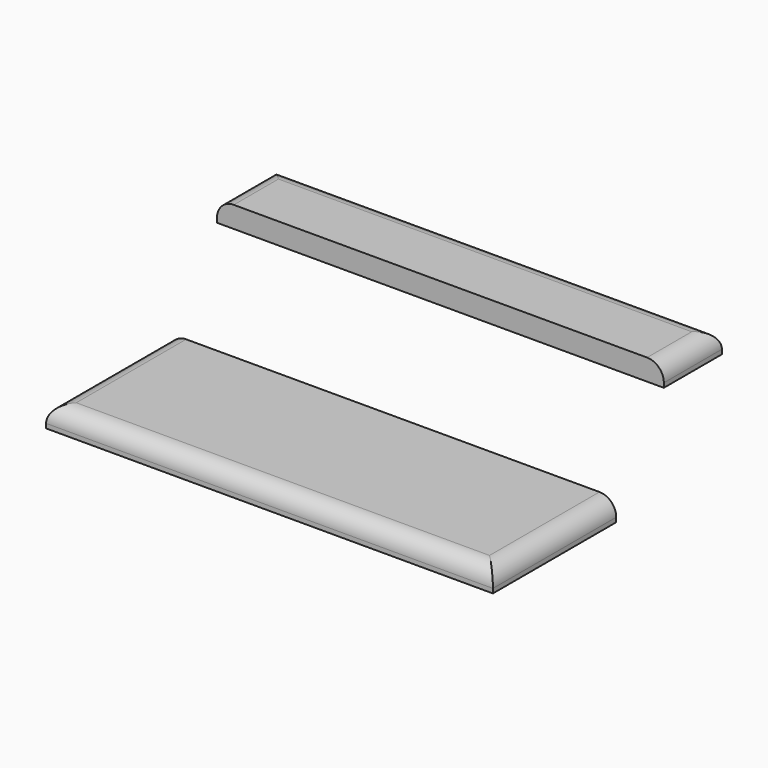
from build123d import *

# Parameters (mm, degrees)
F1_W     = 400
F1_H     = 65
F2_DEPTH = 19
F0_W     = 400
F0_H     = 138
F3_DEPTH = 19
F4_R     = 15
F4_2_R   = 15


with BuildPart() as f2:
    # F1 (on Top) → F2 (new body)
    with BuildSketch(Plane.XY):
        with Locations((-200, 277.2595660102)):
            Rectangle(F1_W, F1_H)
    extrude(amount=F2_DEPTH)

    # F4
    f4_edges = [f2.edges().sort_by_distance(p)[0] for p in [
        (-200, 309.759566, 19),
        (-400, 277.259566, 19),
        (0, 277.259566, 19),
    ]]
    fillet(f4_edges, radius=F4_R)


with BuildPart() as f3:
    # F0 (on Top) → F3 (new body)
    with BuildSketch(Plane.XY):
        with Locations((-98.8323359787, -3.9581097662)):
            Rectangle(F0_W, F0_H)
    extrude(amount=F3_DEPTH)

    # F4#2
    f4_2_edges = [f3.edges().sort_by_distance(p)[0] for p in [
        (-98.832336, -72.95811, 19),
        (-298.832336, -3.95811, 19),
        (101.167664, -3.95811, 19),
    ]]
    fillet(f4_2_edges, radius=F4_2_R)


solid = Compound([f2.part, f3.part])
